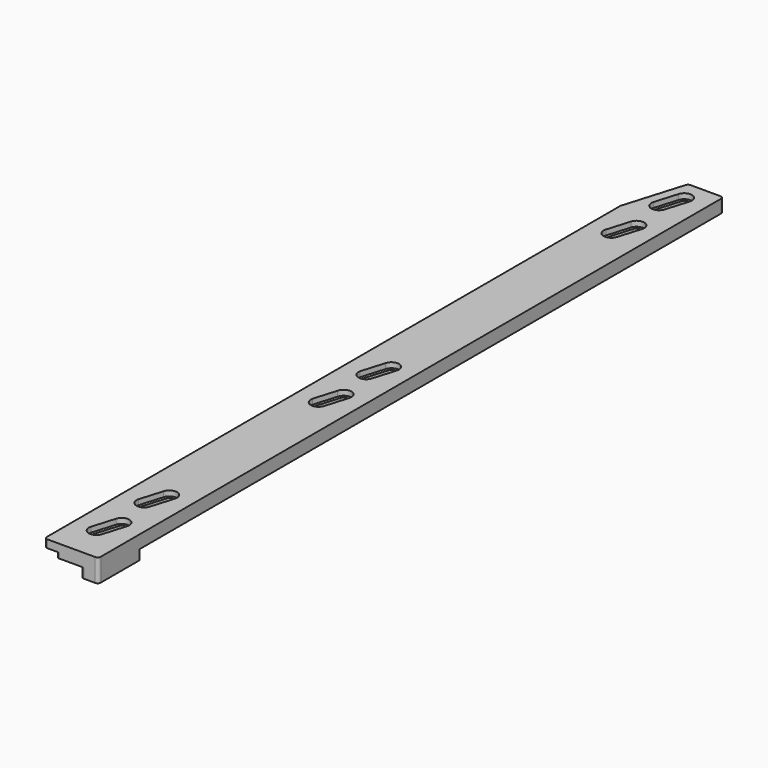
from build123d import *

# Parameters (mm, degrees)
F1_DEPTH    = 4.25
F2_W        = 3.9
F2_H        = 25.4
F3_DEPTH    = 1.7
F4_DEPTH    = 3.165
F5_R        = 1
F6_T1_DEPTH = 11.6817943787
F8_DEPTH    = 1.7
F9_DEPTH    = 25


# Not quite as in the source:
# - a fillet or chamfer that OpenCascade refuses, or shapes differently, is made with other operations: its cross-section is extruded or revolved along the edge and cut away or added
# - a feature names something its author has since deleted; it is built from what else it names


with BuildPart() as f1:
    # F0 (on Top) → F1 (new body)
    with BuildSketch(Plane.XY):
        Polygon((8.75, 106.9650896668), (-2.75, 106.9650896668), (-8.75, 86.9647799072), (-8.75, -147.0349103332), (8.75, -147.0349103332), align=None)
    extrude(amount=-F1_DEPTH)

    # F2 (on face) → F3 (cut)
    with BuildSketch(Plane(origin=(0, 0, -4.25), x_dir=(1, 0, 0), z_dir=(0, 0, -1))):
        with Locations((-6.8, 134.3349103332)):
            Rectangle(F2_W, F2_H)
        Polygon((-8.75, 78.5952200928), (-8.75, 58.5949103332), (-2.75, 58.5949103332), align=None)
        Polygon((-8.75, -4.1847799072), (-8.75, -24.1850896668), (-2.75, -24.1850896668), align=None)
    extrude(amount=-F3_DEPTH, mode=Mode.SUBTRACT)

    # F2 (on face) → F4 (join)
    with BuildSketch(Plane(origin=(0, 0, -4.25), x_dir=(1, 0, 0), z_dir=(0, 0, -1))):
        Polygon((2.75, 147.0349103332), (8.75, 127.0349103332), (8.75, 147.0349103332), align=None)
    extrude(amount=F4_DEPTH)

    # F5
    f5_edges = [f1.edges().sort_by_distance(p)[0] for p in [
        (-2.75, -58.59491, -3.4),
        (-8.75, -58.59491, -3.4),
        (-4.85, -121.63491, -3.4),
        (-8.75, -121.63491, -3.4),
        (-4.85, -147.03491, -3.4),
        (-8.75, -147.03491, -1.275),
        (8.75, -147.03491, -3.7075),
        (2.75, -147.03491, -5.8325),
        (-2.75, 24.18509, -3.4),
        (-8.75, 24.18509, -3.4),
        (8.75, 106.96509, -2.125),
        (-2.75, 106.96509, -2.125),
    ]]
    fillet(f5_edges, radius=F5_R)

    # F6: fillet of radius 0.5 on 1 edges, made by hand

    # F6_s2 → F6_t1 (cut)
    with BuildSketch(Plane.XY.offset(-15.9317943787)):
        with BuildLine():
            ThreePointArc((8.75, -130.4416280846), (8.3226065723, -129.9469278869), (7.7710868574, -130.2979541419))
            Line((7.7710868574, -130.2979541419), (8.75, -127.0349103332))
            Line((8.75, -127.0349103332), (8.75, -130.4416280846))
        make_face()
    extrude(amount=F6_T1_DEPTH, mode=Mode.SUBTRACT)

    # F7 (on face) → F8 (cut)
    with BuildSketch(Plane.XY):
        with BuildLine():
            Line((-1.281113759, 101.2524492275), (-3.5080282296, 93.8292860243))
            ThreePointArc((-3.5080282296, 93.8292860243), (-1.8318189791, 90.7163576177), (1.2811093315, 92.3925670464))
            Line((1.2811093315, 92.3925670464), (3.508023802, 99.8157302495))
            ThreePointArc((3.508023802, 99.8157302495), (1.831814489, 102.9286584474), (-1.281113759, 101.2524492275))
        make_face()
        with BuildLine():
            Line((2.5501962221, 100.1030738196), (0.3232817516, 92.6799106164))
            ThreePointArc((0.3232817516, 92.6799106164), (-1.5444751953, 91.6741851335), (-2.5502007779, 93.5419420268))
            Line((-2.5502007779, 93.5419420268), (-0.3232863074, 100.9651052299))
            ThreePointArc((-0.3232863074, 100.9651052299), (1.5444707052, 101.9708309316), (2.5501962221, 100.1030738196))
        make_face(mode=Mode.SUBTRACT)
        with BuildLine():
            Line((-1.281113759, 81.8682859589), (-3.5080282296, 74.4451227557))
            ThreePointArc((-3.5080282296, 74.4451227557), (-1.8318189791, 71.3321943492), (1.2811093315, 73.0084037778))
            Line((1.2811093315, 73.0084037778), (3.508023802, 80.431566981))
            ThreePointArc((3.508023802, 80.431566981), (1.831814489, 83.5444951788), (-1.281113759, 81.8682859589))
        make_face()
        with BuildLine():
            Line((2.5501962221, 80.718910551), (0.3232817516, 73.2957473478))
            ThreePointArc((0.3232817516, 73.2957473478), (-1.5444751953, 72.2900218649), (-2.5502007779, 74.1577787582))
            Line((-2.5502007779, 74.1577787582), (-0.3232863074, 81.5809419614))
            ThreePointArc((-0.3232863074, 81.5809419614), (1.5444707052, 82.586667663), (2.5501962221, 80.718910551))
        make_face(mode=Mode.SUBTRACT)
        with BuildLine():
            Line((-1.3184834487, -37.2262845319), (-3.5453934487, -44.6494328331))
            ThreePointArc((-3.5453934487, -44.6494328331), (-1.6928299922, -47.6607462741), (1.3184834487, -45.8081828176))
            Line((1.3184834487, -45.8081828176), (3.5453934487, -38.3850345164))
            ThreePointArc((3.5453934487, -38.3850345164), (1.6928299922, -35.3737210755), (-1.3184834487, -37.2262845319))
        make_face()
        with BuildLine():
            ThreePointArc((-0.32342291, -37.3750995728), (1.5027069877, -36.3570453968), (2.5726180692, -38.1532845195))
            Line((2.5726180692, -38.1532845195), (0.3457080692, -45.5764328207))
            ThreePointArc((0.3457080692, -45.5764328207), (-1.4610799953, -46.6879708946), (-2.5726180692, -44.88118283))
            Line((-2.5726180692, -44.88118283), (-0.32342291, -37.3750995728))
        make_face(mode=Mode.SUBTRACT)
        with BuildLine():
            ThreePointArc((-3.5453934487, -25.2652845319), (-1.6928299922, -28.2765979729), (1.3184834487, -26.4240345164))
            Line((1.3184834487, -26.4240345164), (3.5453979193, -19.0008713133))
            ThreePointArc((3.5453979193, -19.0008713133), (1.6928344628, -15.9895578723), (-1.3184789782, -17.8421213288))
            Line((-1.3184789782, -17.8421213288), (-3.5453934487, -25.2652845319))
        make_face()
        with BuildLine():
            ThreePointArc((0.3513294529, -26.167779481), (-1.4365749568, -27.3094439771), (-2.5782394529, -25.5215395674))
            Line((-2.5782394529, -25.5215395674), (-0.3513249813, -18.0983763605))
            ThreePointArc((-0.3513249813, -18.0983763605), (1.4365749587, -16.9567321352), (2.5782439235, -18.7446162778))
            Line((2.5782439235, -18.7446162778), (0.3513294529, -26.167779481))
        make_face(mode=Mode.SUBTRACT)
        with BuildLine():
            Line((-1.2811093046, -107.9180212426), (-3.5080237752, -115.3411844458))
            ThreePointArc((-3.5080237752, -115.3411844458), (-1.8318145066, -118.4541127276), (1.2811137752, -116.7779034591))
            Line((1.2811137752, -116.7779034591), (3.5080282457, -109.3547402559))
            ThreePointArc((3.5080282457, -109.3547402559), (1.8318145067, -106.2418268761), (-1.2811093046, -107.9180212426))
        make_face()
        with BuildLine():
            ThreePointArc((-0.3232817945, -108.2053650453), (1.544470704, -107.1996543861), (2.5502007356, -109.0673964532))
            Line((2.5502007356, -109.0673964532), (0.3232862651, -116.4905596564))
            ThreePointArc((0.3232862651, -116.4905596564), (-1.544470704, -117.4962852176), (-2.5501962651, -115.6285282484))
            Line((-2.5501962651, -115.6285282484), (-0.3232817945, -108.2053650453))
        make_face(mode=Mode.SUBTRACT)
        with BuildLine():
            Line((-1.280113287, -127.2988486416), (-3.507023287, -134.7220131859))
            ThreePointArc((-3.507023287, -134.7220131859), (-1.8036595485, -137.8465346478), (1.2982333531, -136.1023033504))
            Line((1.2982333531, -136.1023033504), (3.5251433531, -128.6791388061))
            ThreePointArc((3.5251433531, -128.6791388061), (1.8036595485, -125.6176994193), (-1.280113287, -127.2988486416))
        make_face()
        with BuildLine():
            ThreePointArc((0.308713365, -135.9206030083), (-1.5472756815, -136.8795961043), (-2.5617754063, -135.0533558662))
            Line((-2.5617754063, -135.0533558662), (-0.3348654063, -127.6301913219))
            ThreePointArc((-0.3348654063, -127.6301913219), (1.5472756815, -126.5846379628), (2.535623365, -128.4974384639))
            Line((2.535623365, -128.4974384639), (0.308713365, -135.9206030083))
        make_face(mode=Mode.SUBTRACT)
    extrude(amount=-F8_DEPTH, mode=Mode.SUBTRACT)

    # F7 (on face) → F9 (cut)
    with BuildSketch(Plane.XY):
        with BuildLine():
            Line((-0.3348654063, -127.6301913219), (-2.5617754063, -135.0533558662))
            ThreePointArc((-2.5617754063, -135.0533558662), (-1.5472756815, -136.8795961043), (0.308713365, -135.9206030083))
            Line((0.308713365, -135.9206030083), (2.535623365, -128.4974384639))
            ThreePointArc((2.535623365, -128.4974384639), (1.5472756815, -126.5846379628), (-0.3348654063, -127.6301913219))
        make_face()
        with BuildLine():
            Line((0.3232862651, -116.4905596564), (2.5502007356, -109.0673964532))
            ThreePointArc((2.5502007356, -109.0673964532), (1.544470704, -107.1996543861), (-0.3232817945, -108.2053650453))
            Line((-0.3232817945, -108.2053650453), (-2.5501962651, -115.6285282484))
            ThreePointArc((-2.5501962651, -115.6285282484), (-1.544470704, -117.4962852176), (0.3232862651, -116.4905596564))
        make_face()
        with BuildLine():
            Line((0.3457080692, -45.5764328207), (2.5726180692, -38.1532845195))
            ThreePointArc((2.5726180692, -38.1532845195), (1.5027069877, -36.3570453968), (-0.32342291, -37.3750995728))
            Line((-0.32342291, -37.3750995728), (-2.5726180692, -44.88118283))
            ThreePointArc((-2.5726180692, -44.88118283), (-1.4610799953, -46.6879708946), (0.3457080692, -45.5764328207))
        make_face()
        with BuildLine():
            Line((-0.3513249813, -18.0983763605), (-2.5782394529, -25.5215395674))
            ThreePointArc((-2.5782394529, -25.5215395674), (-1.4365749568, -27.3094439771), (0.3513294529, -26.167779481))
            Line((0.3513294529, -26.167779481), (2.5782439235, -18.7446162778))
            ThreePointArc((2.5782439235, -18.7446162778), (1.4365749587, -16.9567321352), (-0.3513249813, -18.0983763605))
        make_face()
        with BuildLine():
            ThreePointArc((-2.5502007779, 93.5419420268), (-1.5444751953, 91.6741851335), (0.3232817516, 92.6799106164))
            Line((0.3232817516, 92.6799106164), (2.5501962221, 100.1030738196))
            ThreePointArc((2.5501962221, 100.1030738196), (1.5444707052, 101.9708309316), (-0.3232863074, 100.9651052299))
            Line((-0.3232863074, 100.9651052299), (-2.5502007779, 93.5419420268))
        make_face()
        with BuildLine():
            ThreePointArc((-2.5502007779, 74.1577787582), (-1.5444751953, 72.2900218649), (0.3232817516, 73.2957473478))
            Line((0.3232817516, 73.2957473478), (2.5501962221, 80.718910551))
            ThreePointArc((2.5501962221, 80.718910551), (1.5444707052, 82.586667663), (-0.3232863074, 81.5809419614))
            Line((-0.3232863074, 81.5809419614), (-2.5502007779, 74.1577787582))
        make_face()
    extrude(amount=-F9_DEPTH, mode=Mode.SUBTRACT)


solid = f1.part
